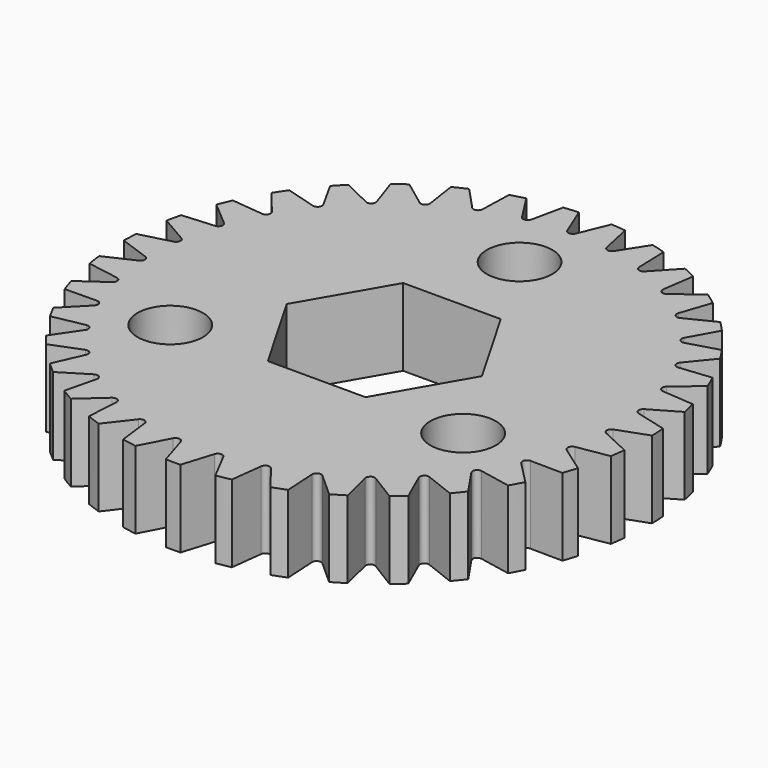
from build123d import *

# Parameters (mm, degrees)
F0_R            = 17.3565013667
F0_R_2          = 2.15265
F1_DEPTH        = 5.08
F3_DEPTH        = 5.08
F3_COPIES_COUNT = 35


# Not quite as in the source:
# - a pattern or mirror of a feature is missing from the dataset's text; its kind, count and spacing are read off the source's solid
# - a feature names something its author has since deleted; it is built from what else it names


with BuildPart() as f1:
    # F0 (on Top) → F1 (new body)
    with BuildSketch(Plane.XY):
        Circle(F0_R)
        with Locations((-9.6237072996, -5.55625)):
            Circle(F0_R_2, mode=Mode.SUBTRACT)
        with Locations((9.6237072996, -5.55625)):
            Circle(F0_R_2, mode=Mode.SUBTRACT)
        Polygon((6.4158048664, 0), (3.2079024332, -5.55625), (-3.2079024332, -5.55625), (-6.4158048664, 0), (-3.2079024332, 5.55625), (3.2079024332, 5.55625), align=None, mode=Mode.SUBTRACT)
        with Locations((0, 11.1125)):
            Circle(F0_R_2, mode=Mode.SUBTRACT)
    extrude(amount=F1_DEPTH)

    # F2 (on face) → F3 (cut, through all)
    with BuildSketch(Plane.XY.offset(5.08)):
        with BuildLine():
            Line((0.275157943, 15.3777549622), (1.0756124971, 17.3231405192))
            ThreePointArc((1.0756124971, 17.3231405192), (0, 17.3565013667), (-1.0756124971, 17.3231405192))
            Line((-1.0756124971, 17.3231405192), (-0.275157943, 15.3777549622))
            ThreePointArc((-0.275157943, 15.3777549622), (0, 15.1934323047), (0.275157943, 15.3777549622))
        make_face()
    f3 = extrude(amount=-F3_DEPTH, mode=Mode.SUBTRACT)

    # F3_copies: F3 ×35 about axis
    f3_copies_axis = Axis((0, 0, 0), (0, 0, 1))
    for i in range(1, F3_COPIES_COUNT):
        add(f3.rotate(f3_copies_axis, i * 360 / F3_COPIES_COUNT), mode=Mode.SUBTRACT)


solid = f1.part
